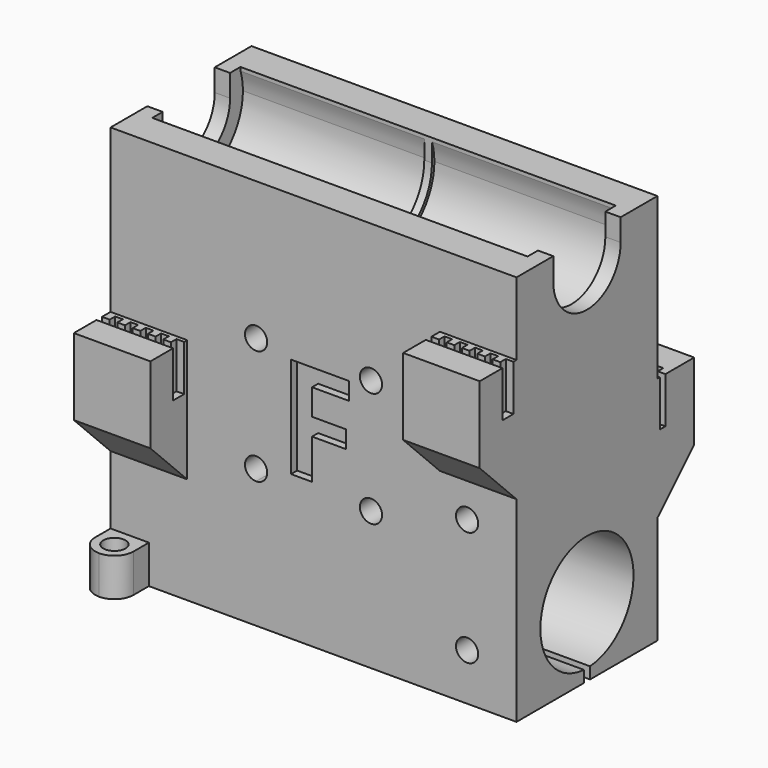
from build123d import *

# Parameters (mm, degrees)
F3_W          = 53
F3_H          = 23
F4_DEPTH      = 51.1
F6_DEPTH      = 53.001
F7_DEPTH      = 51
F8_DEPTH      = 27
F9_DEPTH      = 26
F10_DEPTH     = 2
F11_W         = 10
F11_H         = 20
F12_DEPTH     = 6
F13_T4_DEPTH  = 61.4336597593
F13_T9_DEPTH  = 61.4336597593
F15_DEPTH     = 6
F17_W         = 10
F17_H         = 20
F18_DEPTH     = 6
F20_DEPTH     = 6
F22_DEPTH     = 6
F23_T4_DEPTH  = 61.4336597593
F23_T9_DEPTH  = 61.4336597593
F24_R         = 1.45
F25_DEPTH     = 29.001
F26_R         = 1.45
F27_DEPTH     = 5
F28_TEXT_SIZE = 18.4411155982
F29_DEPTH     = 1
F30_W         = 5
F30_H         = 5
F31_DEPTH     = 5
F33_DEPTH     = 25
F34_R         = 2.49999
F35_DEPTH     = 6


# Not quite as in the source:
# - a fillet or chamfer that OpenCascade refuses, or shapes differently, is made with other operations: its cross-section is extruded or revolved along the edge and cut away or added
# - a fillet or chamfer is up to 0.001 mm smaller than in the source, because OpenCascade refuses the exact size
# - a feature names something its author has since deleted; it is built from what else it names
# - Text() gives the source's letters only with a copy of the font that has no kerning and outlines rounded to 1/6400 em; it was checked with that copy


with BuildPart() as f4:
    # F3 (on Top) → F4 (new body)
    with BuildSketch(Plane.XY):
        with Locations((26.5, 11.5)):
            Rectangle(F3_W, F3_H)
    extrude(amount=F4_DEPTH)

    # F5 (on face) → F6 (cut, through all)
    with BuildSketch(Plane(origin=(0, 0, 0), x_dir=(0, -1, 0), z_dir=(-1, 0, 0))):
        with BuildLine():
            Line((-11.5, 15.5999502167), (-6.9974287961, 15.2226507784))
            ThreePointArc((-6.9974287961, 15.2226507784), (-9.1306272893, 16.3212237853), (-11.5, 16.7))
            Line((-11.5, 16.7), (-11.5, 15.5999502167))
        make_face()
        with BuildLine():
            Line((-11.5, 15.5999502167), (-11.5, 16.7))
            ThreePointArc((-11.5, 16.7), (-13.8693727107, 16.3212237853), (-16.0025712039, 15.2226507784))
            Line((-16.0025712039, 15.2226507784), (-11.5, 15.5999502167))
        make_face()
        with BuildLine():
            Line((-11, 0), (-11, 1.5164652041))
            ThreePointArc((-11, 1.5164652041), (-11.5, 1.5), (-12, 1.5164652041))
            Line((-12, 1.5164652041), (-12, 0))
            Line((-12, 0), (-11.5, 0))
            Line((-11.5, 0), (-11, 0))
        make_face()
        with BuildLine():
            ThreePointArc((-12, 1.5164652041), (-11.5, 1.5), (-11, 1.5164652041))
            Line((-11, 1.5164652041), (-12, 1.5164652041))
        make_face()
        with BuildLine():
            ThreePointArc((-11, 1.5164652041), (-5.9520273973, 3.9057724347), (-3.9, 9.1))
            ThreePointArc((-3.9, 9.1), (-4.718424182, 12.5307767962), (-6.9974287961, 15.2226507784))
            Line((-6.9974287961, 15.2226507784), (-11.5, 15.5999502167))
            Line((-11.5, 15.5999502167), (-16.0025712039, 15.2226507784))
            ThreePointArc((-16.0025712039, 15.2226507784), (-18.7952937166, 6.9695799502), (-12, 1.5164652041))
            Line((-12, 1.5164652041), (-11, 1.5164652041))
        make_face()
        with BuildLine():
            Line((-6, 48.2), (-6, 51.1))
            Line((-6, 51.1), (-6.8266714218, 51.1))
            ThreePointArc((-6.8266714218, 51.1), (-6.2107038663, 49.7077620535), (-6, 48.2))
        make_face()
        with BuildLine():
            Line((-16.1733285782, 51.1), (-17, 51.1))
            Line((-17, 51.1), (-17, 48.2))
            ThreePointArc((-17, 48.2), (-16.7892961337, 49.7077620535), (-16.1733285782, 51.1))
        make_face()
        with BuildLine():
            ThreePointArc((-17, 48.2), (-11.5, 42.7), (-6, 48.2))
            ThreePointArc((-6, 48.2), (-6.2107038663, 49.7077620535), (-6.8266714218, 51.1))
            Line((-6.8266714218, 51.1), (-16.1733285782, 51.1))
            ThreePointArc((-16.1733285782, 51.1), (-16.7892961337, 49.7077620535), (-17, 48.2))
        make_face()
    extrude(amount=-F6_DEPTH, mode=Mode.SUBTRACT)

    # F5 (on face) → F7 (cut)
    with BuildSketch(Plane(origin=(0, 0, 0), x_dir=(0, -1, 0), z_dir=(-1, 0, 0))):
        with BuildLine():
            ThreePointArc((-18.7, 48.2), (-11.5, 41), (-4.3, 48.2))
            ThreePointArc((-4.3, 48.2), (-4.4541133303, 49.6817155724), (-4.9098558438, 51.1))
            Line((-4.9098558438, 51.1), (-6, 51.1))
            Line((-6, 51.1), (-6, 48.2))
            ThreePointArc((-6, 48.2), (-11.5, 42.7), (-17, 48.2))
            Line((-17, 48.2), (-17, 51.1))
            Line((-17, 51.1), (-18.0901441562, 51.1))
            ThreePointArc((-18.0901441562, 51.1), (-18.5458866697, 49.6817155724), (-18.7, 48.2))
        make_face()
        with BuildLine():
            Line((-4.3, 48.2), (-4.3, 50.6331050121))
            ThreePointArc((-4.3, 50.6331050121), (-4.3836921378, 50.8679884577), (-4.4750444841, 51.1))
            Line((-4.4750444841, 51.1), (-4.9098558438, 51.1))
            ThreePointArc((-4.9098558438, 51.1), (-4.4541133303, 49.6817155724), (-4.3, 48.2))
        make_face()
        with BuildLine():
            ThreePointArc((-18.5249555159, 51.1), (-18.6163078622, 50.8679884577), (-18.7, 50.6331050121))
            Line((-18.7, 50.6331050121), (-18.7, 48.2))
            ThreePointArc((-18.7, 48.2), (-18.5458866697, 49.6817155724), (-18.0901441562, 51.1))
            Line((-18.0901441562, 51.1), (-18.5249555159, 51.1))
        make_face()
        with BuildLine():
            Line((-18.5249555159, 51.1), (-18.7, 51.1))
            Line((-18.7, 51.1), (-18.7, 50.6331050121))
            ThreePointArc((-18.7, 50.6331050121), (-18.6163078622, 50.8679884577), (-18.5249555159, 51.1))
        make_face()
        with BuildLine():
            ThreePointArc((-19.1, 48.2), (-11.5, 40.6), (-3.9, 48.2))
            ThreePointArc((-3.9, 48.2), (-4.0006666963, 49.4328828006), (-4.3, 50.6331050121))
            Line((-4.3, 50.6331050121), (-4.3, 48.2))
            ThreePointArc((-4.3, 48.2), (-11.5, 41), (-18.7, 48.2))
            Line((-18.7, 48.2), (-18.7, 50.6331050121))
            ThreePointArc((-18.7, 50.6331050121), (-18.9993333037, 49.4328828006), (-19.1, 48.2))
        make_face()
        with BuildLine():
            Line((-4.3, 50.6331050121), (-4.3, 51.1))
            Line((-4.3, 51.1), (-4.4750444841, 51.1))
            ThreePointArc((-4.4750444841, 51.1), (-4.3836921378, 50.8679884577), (-4.3, 50.6331050121))
        make_face()
    extrude(amount=-F7_DEPTH, mode=Mode.SUBTRACT)

    # F5 (on face) → F8 (join)
    with BuildSketch(Plane(origin=(0, 0, 0), x_dir=(0, -1, 0), z_dir=(-1, 0, 0))):
        with BuildLine():
            ThreePointArc((-19.1, 48.2), (-11.5, 40.6), (-3.9, 48.2))
            ThreePointArc((-3.9, 48.2), (-4.0006666963, 49.4328828006), (-4.3, 50.6331050121))
            Line((-4.3, 50.6331050121), (-4.3, 48.2))
            ThreePointArc((-4.3, 48.2), (-11.5, 41), (-18.7, 48.2))
            Line((-18.7, 48.2), (-18.7, 50.6331050121))
            ThreePointArc((-18.7, 50.6331050121), (-18.9993333037, 49.4328828006), (-19.1, 48.2))
        make_face()
    extrude(amount=-F8_DEPTH)

    # F5 (on face) → F9 (cut)
    with BuildSketch(Plane(origin=(0, 0, 0), x_dir=(0, -1, 0), z_dir=(-1, 0, 0))):
        with BuildLine():
            ThreePointArc((-18.7, 48.2), (-11.5, 41), (-4.3, 48.2))
            ThreePointArc((-4.3, 48.2), (-4.4541133303, 49.6817155724), (-4.9098558438, 51.1))
            Line((-4.9098558438, 51.1), (-6, 51.1))
            Line((-6, 51.1), (-6, 48.2))
            ThreePointArc((-6, 48.2), (-11.5, 42.7), (-17, 48.2))
            Line((-17, 48.2), (-17, 51.1))
            Line((-17, 51.1), (-18.0901441562, 51.1))
            ThreePointArc((-18.0901441562, 51.1), (-18.5458866697, 49.6817155724), (-18.7, 48.2))
        make_face()
        with BuildLine():
            Line((-4.3, 50.6331050121), (-4.3, 51.1))
            Line((-4.3, 51.1), (-4.4750444841, 51.1))
            ThreePointArc((-4.4750444841, 51.1), (-4.3836921378, 50.8679884577), (-4.3, 50.6331050121))
        make_face()
        with BuildLine():
            Line((-18.5249555159, 51.1), (-18.7, 51.1))
            Line((-18.7, 51.1), (-18.7, 50.6331050121))
            ThreePointArc((-18.7, 50.6331050121), (-18.6163078622, 50.8679884577), (-18.5249555159, 51.1))
        make_face()
        with BuildLine():
            ThreePointArc((-19.1, 48.2), (-11.5, 40.6), (-3.9, 48.2))
            ThreePointArc((-3.9, 48.2), (-4.0006666963, 49.4328828006), (-4.3, 50.6331050121))
            Line((-4.3, 50.6331050121), (-4.3, 48.2))
            ThreePointArc((-4.3, 48.2), (-11.5, 41), (-18.7, 48.2))
            Line((-18.7, 48.2), (-18.7, 50.6331050121))
            ThreePointArc((-18.7, 50.6331050121), (-18.9993333037, 49.4328828006), (-19.1, 48.2))
        make_face()
        with BuildLine():
            ThreePointArc((-18.5249555159, 51.1), (-18.6163078622, 50.8679884577), (-18.7, 50.6331050121))
            Line((-18.7, 50.6331050121), (-18.7, 48.2))
            ThreePointArc((-18.7, 48.2), (-18.5458866697, 49.6817155724), (-18.0901441562, 51.1))
            Line((-18.0901441562, 51.1), (-18.5249555159, 51.1))
        make_face()
        with BuildLine():
            Line((-16.1733285782, 51.1), (-17, 51.1))
            Line((-17, 51.1), (-17, 48.2))
            ThreePointArc((-17, 48.2), (-16.7892961337, 49.7077620535), (-16.1733285782, 51.1))
        make_face()
        with BuildLine():
            Line((-4.3, 48.2), (-4.3, 50.6331050121))
            ThreePointArc((-4.3, 50.6331050121), (-4.3836921378, 50.8679884577), (-4.4750444841, 51.1))
            Line((-4.4750444841, 51.1), (-4.9098558438, 51.1))
            ThreePointArc((-4.9098558438, 51.1), (-4.4541133303, 49.6817155724), (-4.3, 48.2))
        make_face()
    extrude(amount=-F9_DEPTH, mode=Mode.SUBTRACT)

    # F5 (on face) → F10 (join)
    with BuildSketch(Plane(origin=(0, 0, 0), x_dir=(0, -1, 0), z_dir=(-1, 0, 0))):
        with BuildLine():
            ThreePointArc((-18.7, 48.2), (-11.5, 41), (-4.3, 48.2))
            ThreePointArc((-4.3, 48.2), (-4.4541133303, 49.6817155724), (-4.9098558438, 51.1))
            Line((-4.9098558438, 51.1), (-6, 51.1))
            Line((-6, 51.1), (-6, 48.2))
            ThreePointArc((-6, 48.2), (-11.5, 42.7), (-17, 48.2))
            Line((-17, 48.2), (-17, 51.1))
            Line((-17, 51.1), (-18.0901441562, 51.1))
            ThreePointArc((-18.0901441562, 51.1), (-18.5458866697, 49.6817155724), (-18.7, 48.2))
        make_face()
        with BuildLine():
            Line((-18.7, 51.1), (-19.1, 51.1))
            Line((-19.1, 51.1), (-19.1, 48.2))
            ThreePointArc((-19.1, 48.2), (-18.9993333037, 49.4328828006), (-18.7, 50.6331050121))
            Line((-18.7, 50.6331050121), (-18.7, 51.1))
        make_face()
        with BuildLine():
            Line((-3.9, 48.2), (-3.9, 51.1))
            Line((-3.9, 51.1), (-4.3, 51.1))
            Line((-4.3, 51.1), (-4.3, 50.6331050121))
            ThreePointArc((-4.3, 50.6331050121), (-4.0006666963, 49.4328828006), (-3.9, 48.2))
        make_face()
        with BuildLine():
            ThreePointArc((-19.1, 48.2), (-11.5, 40.6), (-3.9, 48.2))
            ThreePointArc((-3.9, 48.2), (-4.0006666963, 49.4328828006), (-4.3, 50.6331050121))
            Line((-4.3, 50.6331050121), (-4.3, 48.2))
            ThreePointArc((-4.3, 48.2), (-11.5, 41), (-18.7, 48.2))
            Line((-18.7, 48.2), (-18.7, 50.6331050121))
            ThreePointArc((-18.7, 50.6331050121), (-18.9993333037, 49.4328828006), (-19.1, 48.2))
        make_face()
        with BuildLine():
            ThreePointArc((-18.5249555159, 51.1), (-18.6163078622, 50.8679884577), (-18.7, 50.6331050121))
            Line((-18.7, 50.6331050121), (-18.7, 48.2))
            ThreePointArc((-18.7, 48.2), (-18.5458866697, 49.6817155724), (-18.0901441562, 51.1))
            Line((-18.0901441562, 51.1), (-18.5249555159, 51.1))
        make_face()
        with BuildLine():
            Line((-18.5249555159, 51.1), (-18.7, 51.1))
            Line((-18.7, 51.1), (-18.7, 50.6331050121))
            ThreePointArc((-18.7, 50.6331050121), (-18.6163078622, 50.8679884577), (-18.5249555159, 51.1))
        make_face()
        with BuildLine():
            Line((-4.3, 48.2), (-4.3, 50.6331050121))
            ThreePointArc((-4.3, 50.6331050121), (-4.3836921378, 50.8679884577), (-4.4750444841, 51.1))
            Line((-4.4750444841, 51.1), (-4.9098558438, 51.1))
            ThreePointArc((-4.9098558438, 51.1), (-4.4541133303, 49.6817155724), (-4.3, 48.2))
        make_face()
        with BuildLine():
            Line((-4.3, 50.6331050121), (-4.3, 51.1))
            Line((-4.3, 51.1), (-4.4750444841, 51.1))
            ThreePointArc((-4.4750444841, 51.1), (-4.3836921378, 50.8679884577), (-4.3, 50.6331050121))
        make_face()
    extrude(amount=-F10_DEPTH)

    # F11 (on face) → F12 (join)
    with BuildSketch(Plane.XZ):
        with Locations((5, 19.9)):
            Rectangle(F11_W, F11_H)
        with Locations((48, 31.6)):
            Rectangle(F11_W, F11_H)
    extrude(amount=F12_DEPTH)

    # F13: chamfer of 10 on 2 edges, made by hand


with BuildPart() as f13_tool2:
    # F13_s3 → F13_t4 (new body)
    with BuildSketch(Plane.YZ.offset(-25.7168298797)):
        Polygon((4, 9.9), (-6, 19.9), (-6, 9.9), align=None)
    extrude(amount=F13_T4_DEPTH)

    split(bisect_by=Plane.XZ, keep=Keep.TOP)


with BuildPart() as f4_1:
    add(f4.part)

    # F13_t1: cut F13_tool2
    add(f13_tool2.part, mode=Mode.SUBTRACT)


with BuildPart() as f13_tool7:
    # F13_s8 → F13_t9 (new body)
    with BuildSketch(Plane.YZ.offset(17.2831701203)):
        Polygon((4, 21.6), (-6, 31.6), (-6, 21.6), align=None)
    extrude(amount=F13_T9_DEPTH)

    split(bisect_by=Plane.XZ, keep=Keep.TOP)


with BuildPart() as f4_2:
    add(f4_1.part)

    # F13_t6: cut F13_tool7
    add(f13_tool7.part, mode=Mode.SUBTRACT)

    # F14 (on face) → F15 (cut)
    with BuildSketch(Plane.XY.offset(29.9)):
        Polygon((0, -1.4), (0, -2.3), (10, -2.3), (10, -1.4), (10, -0.5), (9, -0.5), (9, -1.4), (8, -1.4), (8, -0.5), (7, -0.5), (7, -1.4), (6, -1.4), (6, -0.5), (5.2958247252, -0.5), (5, -0.5), (5, -1.4), (4, -1.4), (4, -0.5), (3, -0.5), (3, -1.4), (2, -1.4), (2, -0.5), (1, -0.5), (1, -1.4), align=None)
    extrude(amount=-F15_DEPTH, mode=Mode.SUBTRACT)

    # F17 (on face) → F18 (join)
    with BuildSketch(Plane(origin=(0, 23, 0), x_dir=(-1, 0, 0), z_dir=(0, 1, 0))):
        with Locations((-48, 20.1)):
            Rectangle(F17_W, F17_H)
        with Locations((-5, 31.6)):
            Rectangle(F17_W, F17_H)
    extrude(amount=F18_DEPTH)

    # F19 (on face) → F20 (cut)
    with BuildSketch(Plane.XY.offset(30.1)):
        Polygon((43, 23.4), (45, 23.4), (46, 23.4), (48, 23.4), (53, 23.4), (53, 24.3), (52, 24.3), (52, 25.2), (51, 25.2), (51, 24.3), (50, 24.3), (50, 25.2), (49, 25.2), (49, 24.3), (48, 24.3), (48, 25.2), (47, 25.2), (47, 24.3), (46, 24.3), (46, 25.2), (45, 25.2), (45, 24.3), (44, 24.3), (44, 25.2), (43, 25.2), align=None)
    extrude(amount=-F20_DEPTH, mode=Mode.SUBTRACT)

    # F21 (on face) → F22 (cut)
    with BuildSketch(Plane.XY.offset(41.6)):
        Polygon((10, 23.4), (10, 25.2), (9, 25.2), (9, 24.3), (8, 24.3), (8, 25.2), (7, 25.2), (7, 24.3), (6, 24.3), (6, 25.2), (5, 25.2), (5, 24.3), (4, 24.3), (4, 25.2), (3, 25.2), (3, 24.3), (2, 24.3), (2, 25.2), (1, 25.2), (1, 24.3), (0, 24.3), (0, 23.4), align=None)
    extrude(amount=-F22_DEPTH, mode=Mode.SUBTRACT)

    # F23: chamfer of 10 on 2 edges, made by hand


with BuildPart() as f23_tool2:
    # F23_s3 → F23_t4 (new body)
    with BuildSketch(Plane.YZ.offset(35.7168298797)):
        Polygon((29, 31.6), (19, 21.6), (29, 21.6), align=None)
    extrude(amount=-F23_T4_DEPTH)

    split(bisect_by=Plane.XZ.offset(-23), keep=Keep.BOTTOM)


with BuildPart() as f4_3:
    add(f4_2.part)

    # F23_t1: cut F23_tool2
    add(f23_tool2.part, mode=Mode.SUBTRACT)


with BuildPart() as f23_tool7:
    # F23_s8 → F23_t9 (new body)
    with BuildSketch(Plane.YZ.offset(78.7168298797)):
        Polygon((19, 10.1), (29, 20.1), (29, 10.1), align=None)
    extrude(amount=-F23_T9_DEPTH)

    split(bisect_by=Plane.XZ.offset(-23), keep=Keep.BOTTOM)


with BuildPart() as f4_4:
    add(f4_3.part)

    # F23_t6: cut F23_tool7
    add(f23_tool7.part, mode=Mode.SUBTRACT)

    # F24 (on face) → F25 (cut, through all)
    with BuildSketch(Plane.XZ):
        with BuildLine():
            ThreePointArc((17.55, 33.05), (19, 31.6), (20.45, 33.05))
            ThreePointArc((20.45, 33.05), (19, 34.5), (17.55, 33.05))
        make_face()
        with BuildLine():
            ThreePointArc((34, 34.5), (32.9746951673, 32.0246951673), (35.45, 33.05))
            ThreePointArc((35.45, 33.05), (35.0253048327, 34.0753048327), (34, 34.5))
        make_face()
        with BuildLine():
            ThreePointArc((19, 16.6), (20.0253048327, 17.0246951673), (20.45, 18.05))
            ThreePointArc((20.45, 18.05), (17.9746951673, 19.0753048327), (19, 16.6))
        make_face()
        with Locations((34, 18.05)):
            Circle(F24_R)
        with BuildLine():
            ThreePointArc((35.45, 33.05), (35.0253048327, 34.0753048327), (34, 34.5))
            ThreePointArc((34, 34.5), (32.9746951673, 32.0246951673), (35.45, 33.05))
        make_face()
        with BuildLine():
            ThreePointArc((20.45, 18.05), (17.9746951673, 19.0753048327), (19, 16.6))
            ThreePointArc((19, 16.6), (20.0253048327, 17.0246951673), (20.45, 18.05))
        make_face()
    extrude(amount=-F25_DEPTH, mode=Mode.SUBTRACT)

    # F26 (on face) → F27 (cut)
    with BuildSketch(Plane.XZ):
        with Locations((46.55, 21.15)):
            Circle(F26_R)
        with Locations((46.55, 6.15)):
            Circle(F26_R)
    extrude(amount=-F27_DEPTH, mode=Mode.SUBTRACT)

    # F28 (on face) → F29 (cut)
    with BuildSketch(Plane.XZ):
        with Locations((21.8983653734, 18.9111983846)):
            Text('F', F28_TEXT_SIZE, font='Open Sans', font_style=FontStyle.BOLD, text_align=(TextAlign.LEFT, TextAlign.BOTTOM))
    extrude(amount=-F29_DEPTH, mode=Mode.SUBTRACT)

    # F30 (on face) → F31 (join)
    with BuildSketch(Plane.XZ):
        with Locations((2.5, 2.5)):
            Rectangle(F30_W, F30_H)
    extrude(amount=F31_DEPTH)

    # F32 (on face) → F33 (cut)
    with BuildSketch(Plane.XY.offset(5)):
        with BuildLine():
            Line((1.05, -2.5), (3.95, -2.5))
            ThreePointArc((3.95, -2.5), (2.5, -1.05), (1.05, -2.5))
        make_face()
        with BuildLine():
            ThreePointArc((1.05, -2.5), (2.5, -3.95), (3.95, -2.5))
            Line((3.95, -2.5), (1.05, -2.5))
        make_face()
    extrude(amount=-F33_DEPTH, mode=Mode.SUBTRACT)

    # F34 (radius 2.5 in the source; OpenCascade refuses exactly that, so slightly less here)
    f34_edges = [f4_4.edges().sort_by_distance(p)[0] for p in [
        (0, -5, 2.5),
        (5, -5, 2.5),
    ]]
    fillet(f34_edges, radius=F34_R)

    # F16 (on face) → F35 (cut)
    with BuildSketch(Plane.XY.offset(41.6)):
        Polygon((43, -1.4), (43, -2.3), (53, -2.3), (53, -1.4), (53, -0.5), (52, -0.5), (52, -1.4), (51, -1.4), (51, -0.5), (50, -0.5), (50, -1.4), (49, -1.4), (49, -0.5), (48.2349036932, -0.5), (48, -0.5), (48, -1.4), (47, -1.4), (47, -0.5), (46, -0.5), (46, -1.4), (45, -1.4), (45, -0.5), (44, -0.5), (44, -1.4), align=None)
    extrude(amount=-F35_DEPTH, mode=Mode.SUBTRACT)


solid = f4_4.part
